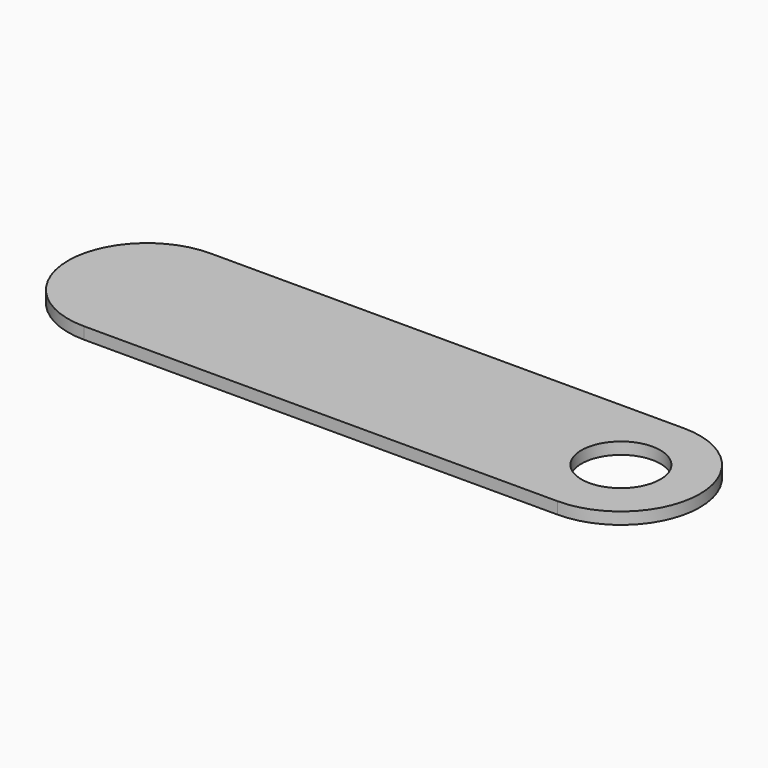
from build123d import *

# Parameters (mm, degrees)
F2_DEPTH = 5.08
F3_R     = 16.9333333333
F4_DEPTH = 5.08
F5_DEPTH = 5.08


# Not quite as in the source:
# - a variable given as a bare number and used for a length is read in inches; the dataset says mm whatever the document's units were


with BuildPart() as f2:
    # F1 (on Top) → F2 (new body)
    with BuildSketch(Plane.XY):
        with BuildLine():
            ThreePointArc((100.8237705737, -47.527355603), (134.6904372404, -13.6606889364), (100.8237705737, 20.2059777303))
            Line((100.8237705737, 20.2059777303), (-102.3762294263, 20.2059777303))
            ThreePointArc((-102.3762294263, 20.2059777303), (-136.2428960929, -13.6606889364), (-102.3762294263, -47.527355603))
            Line((-102.3762294263, -47.527355603), (100.8237705737, -47.527355603))
        make_face()
    extrude(amount=F2_DEPTH)

    # F3 (on face) → F4 (join)
    with BuildSketch(Plane(origin=(0, 0, 0), x_dir=(1, 0, 0), z_dir=(0, 0, -1))):
        with Locations((-102.3762294263, 13.6606889364)):
            Circle(F3_R)
    extrude(amount=F4_DEPTH)

    # F3 (on face) → F5 (cut)
    with BuildSketch(Plane(origin=(0, 0, 0), x_dir=(1, 0, 0), z_dir=(0, 0, -1))):
        with Locations((100.8237705737, 13.6606889364)):
            Circle(F3_R)
    extrude(amount=-F5_DEPTH, mode=Mode.SUBTRACT)


solid = f2.part
